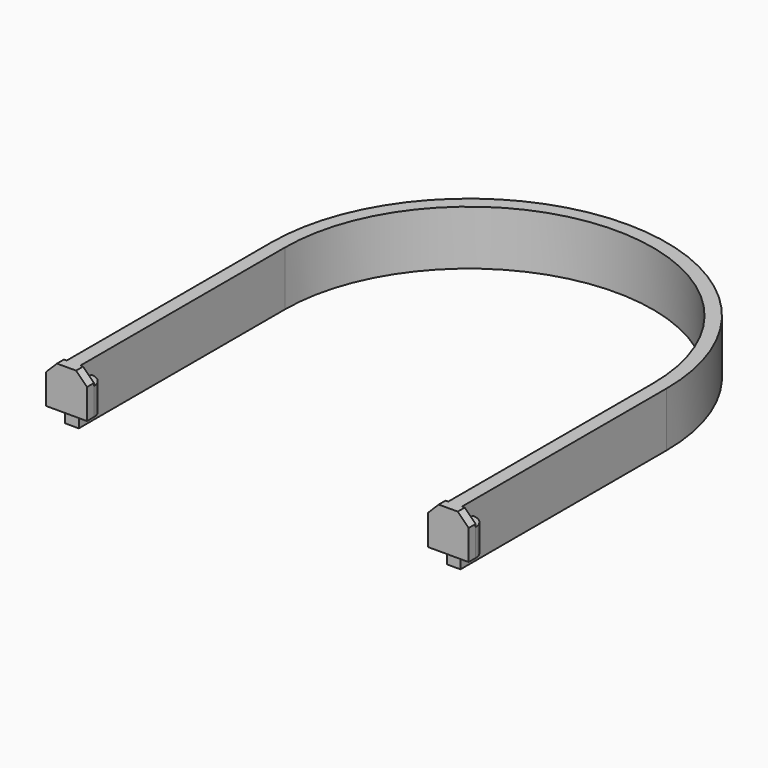
from build123d import *

# Parameters (mm, degrees)
F0_W        = 5
F0_H        = 5
F1_DEPTH    = 20
F2_W        = 2.1819349527
F2_H        = 1.0583491623
F3_DEPTH    = 0.001
F5_DEPTH    = 5
F6_T1_DEPTH = 35
F6_T6_DEPTH = 35
F7_W        = 15
F7_H        = 3.1949503422
F8_DEPTH    = 5
F9_W        = 15
F9_H        = 3.1949481368
F10_DEPTH   = 5
F11_SIZE    = 4


# Not quite as in the source:
# - a fillet or chamfer that OpenCascade refuses, or shapes differently, is made with other operations: its cross-section is extruded or revolved along the edge and cut away or added


with BuildPart() as f1:
    # F0 (on Top) → F1 (new body)
    with BuildSketch(Plane.XY):
        with Locations((-70, -92)):
            Rectangle(F0_W, F0_H)
        with Locations((70, -92)):
            Rectangle(F0_W, F0_H)
        with BuildLine():
            Line((-67.5, -89.5), (-67.5, -26.4575131106))
            ThreePointArc((-67.5, -26.4575131106), (-71.2390342439, -13.4629120178), (-72.5, 0))
            Line((-72.5, 0), (-72.5, -89.5))
            Line((-72.5, -89.5), (-67.5, -89.5))
        make_face()
        with BuildLine():
            ThreePointArc((72.5, 0), (71.2390342439, -13.4629120178), (67.5, -26.4575131106))
            Line((67.5, -26.4575131106), (67.5, -89.5))
            Line((67.5, -89.5), (72.5, -89.5))
            Line((72.5, -89.5), (72.5, 0))
        make_face()
        with BuildLine():
            ThreePointArc((-67.5, 0), (0, 67.5), (67.5, 0))
            Line((67.5, 0), (67.5, -26.4575131106))
            ThreePointArc((67.5, -26.4575131106), (71.2390342439, -13.4629120178), (72.5, 0))
            ThreePointArc((72.5, 0), (0, 72.5), (-72.5, 0))
            ThreePointArc((-72.5, 0), (-71.2390342439, -13.4629120178), (-67.5, -26.4575131106))
            Line((-67.5, -26.4575131106), (-67.5, 0))
        make_face()
    extrude(amount=F1_DEPTH)

    # F2 (on face) → F3 (join)
    with BuildSketch(Plane(origin=(-72.5, 0, 0), x_dir=(0, -1, 0), z_dir=(-1, 0, 0))):
        with Locations((48.3409674764, 10.5291745812)):
            Rectangle(F2_W, F2_H)
    extrude(amount=F3_DEPTH)

    # F4 (on face) → F5 (join, symmetric)
    with BuildSketch(Plane(origin=(0, 0, 10), x_dir=(1, 0, 0), z_dir=(0, 0, -1))):
        Polygon((-67.5, 94.5), (-72.5, 94.5), (-77.5, 94.5), (-77.5, 88.8050496578), (-62.5, 88.8050496578), (-62.5, 94.5), align=None)
        Polygon((-77.5, 94.5), (-72.5, 94.5), (-67.5, 94.5), (-62.5, 94.5), (-62.5, 97), (-77.5, 97), align=None)
        Polygon((72.5142157078, 94.4999977946), (67.5142157078, 94.4999977946), (62.5142157078, 94.4999977946), (62.5142157078, 88.8050496578), (77.5142157078, 88.8050496578), (77.5142157078, 94.4999977946), align=None)
        Polygon((62.5142157078, 94.4999977946), (67.5142157078, 94.4999977946), (72.5142157078, 94.4999977946), (77.5142157078, 94.4999977946), (77.5142157078, 96.9999977946), (62.5142157078, 96.9999977946), align=None)
    extrude(amount=F5_DEPTH, both=True)

    # F6: fillet of radius 5 on 4 edges, made by hand

    # F6_s2 → F6_t1 (cut)
    with BuildSketch(Plane.XY.offset(-7.5)):
        with BuildLine():
            ThreePointArc((-77.5, -93.8050496578), (-76.0355339059, -90.2695157519), (-72.5, -88.8050496578))
            Line((-72.5, -88.8050496578), (-77.5, -88.8050496578))
            Line((-77.5, -88.8050496578), (-77.5, -93.8050496578))
        make_face()
        with BuildLine():
            ThreePointArc((72.5142157078, -88.8050496578), (76.0497496137, -90.2695157519), (77.5142157078, -93.8050496578))
            Line((77.5142157078, -93.8050496578), (77.5142157078, -88.8050496578))
            Line((77.5142157078, -88.8050496578), (72.5142157078, -88.8050496578))
        make_face()
        with BuildLine():
            ThreePointArc((-67.5, -88.8050496578), (-63.9644660941, -90.2695157519), (-62.5, -93.8050496578))
            Line((-62.5, -93.8050496578), (-62.5, -88.8050496578))
            Line((-62.5, -88.8050496578), (-67.5, -88.8050496578))
        make_face()
    extrude(amount=F6_T1_DEPTH, mode=Mode.SUBTRACT)


with BuildPart() as f6_tool4:
    # F6_s5 → F6_t6 (new body)
    with BuildSketch(Plane.XY.offset(-7.5)):
        with BuildLine():
            ThreePointArc((67.5142157078, -88.8050496578), (63.9786818018, -90.2695157519), (62.5142157078, -93.8050496578))
            Line((62.5142157078, -93.8050496578), (62.5142157078, -88.8050496578))
            Line((62.5142157078, -88.8050496578), (67.5142157078, -88.8050496578))
        make_face()
    extrude(amount=F6_T6_DEPTH)

    split(bisect_by=Plane.YZ.offset(67.5), keep=Keep.BOTTOM)


with BuildPart() as f1_1:
    add(f1.part)

    # F6_t3: cut F6_tool4
    add(f6_tool4.part, mode=Mode.SUBTRACT)

    # F7 (on face) → F8 (join)
    with BuildSketch(Plane.XY.offset(15)):
        with Locations((-70, -95.4025248289)):
            Rectangle(F7_W, F7_H)
    extrude(amount=F8_DEPTH)

    # F9 (on face) → F10 (join)
    with BuildSketch(Plane.XY.offset(15)):
        with Locations((70.0142157078, -95.4025237262)):
            Rectangle(F9_W, F9_H)
    extrude(amount=F10_DEPTH)

    # F11
    f11_edges = [f1_1.edges().sort_by_distance(p)[0] for p in [
        (-77.5, -95.402525, 20),
        (62.514216, -95.402524, 20),
        (-62.5, -95.402525, 20),
        (77.514216, -95.402524, 20),
    ]]
    chamfer(f11_edges, length=F11_SIZE)


solid = f1_1.part
